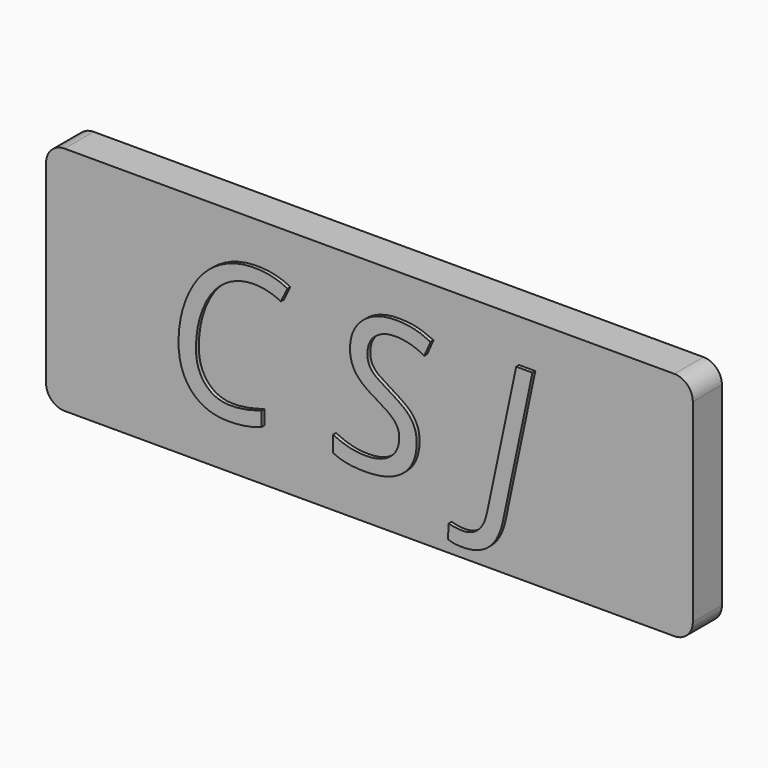
from build123d import *

# Parameters (mm, degrees)
F0_W         = 177.8
F0_H         = 63.5
F1_DEPTH     = 10
F2_R         = 5.08
F3_TEXT_SIZE = 53.7701623721
F4_DEPTH     = 1
F5_TEXT_SIZE = 13.8050177124
F6_DEPTH     = 1


# Not quite as in the source:
# - Text() gives the source's letters only with a copy of the font that has no kerning and outlines rounded to 1/6400 em; it was checked with that copy


with BuildPart() as f1:
    # F0 (on Front) → F1 (new body)
    with BuildSketch(Plane.XZ):
        Rectangle(F0_W, F0_H)
    extrude(amount=F1_DEPTH)

    # F2
    f2_edges = [f1.edges().sort_by_distance(p)[0] for p in [
        (88.9, -5, 31.75),
        (88.9, -5, -31.75),
        (-88.9, -5, -31.75),
        (-88.9, -5, 31.75),
    ]]
    fillet(f2_edges, radius=F2_R)

    # F3 (on face) → F4 (join)
    with BuildSketch(Plane.XZ.offset(10)):
        with Locations((-55.6192640215, -18.3742009103)):
            Text('C S J', F3_TEXT_SIZE, font='Open Sans', font_style=FontStyle.ITALIC, text_align=(TextAlign.LEFT, TextAlign.BOTTOM))
    extrude(amount=F4_DEPTH)

    # F5 (on face) → F6 (join)
    with BuildSketch(Plane(origin=(0, 0, 0), x_dir=(-1, 0, 0), z_dir=(0, 1, 0))):
        with Locations((-44.2996196018, -3.6674906602)):
            Text('heros of storm', F5_TEXT_SIZE, font='Open Sans', font_style=FontStyle.ITALIC, text_align=(TextAlign.LEFT, TextAlign.BOTTOM))
    extrude(amount=F6_DEPTH)


solid = f1.part
